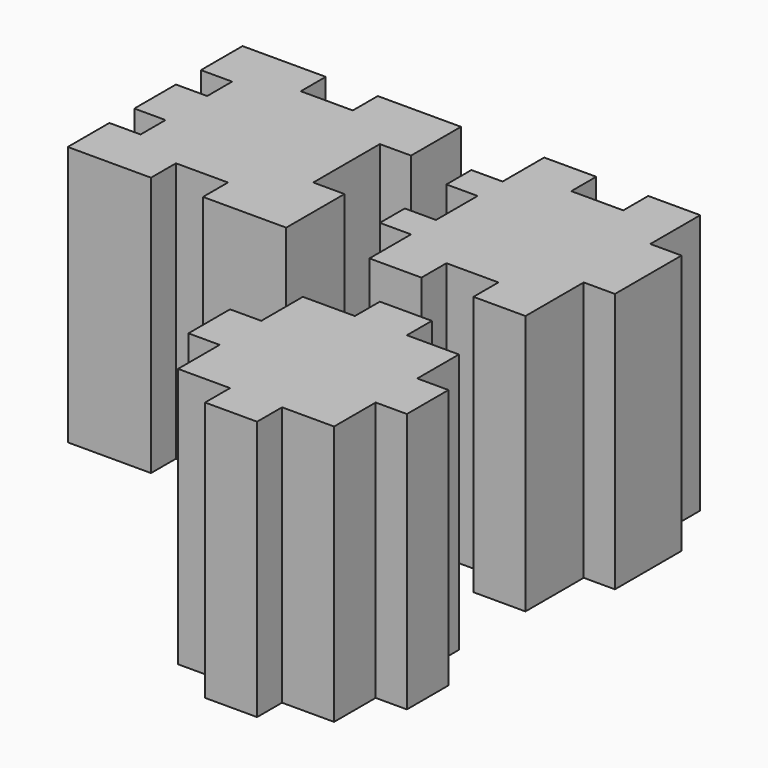
from build123d import *

# Parameters (mm, degrees)
F1_DEPTH = 25


# Not quite as in the source:
# - a feature names something its author has since deleted; it is built from what else it names


with BuildPart() as f1:
    # F0 (on Top) → F1 (new body)
    with BuildSketch(Plane.XY):
        Polygon((10.5, 10.5), (5.5, 10.5), (5.5, 5.5), (2.5, 5.5), (2.5, 2.5), (5.5, 2.5), (5.5, -2.5), (2.5, -2.5), (2.5, -5.5), (5.5, -5.5), (5.5, -10.5), (10.5, -10.5), (10.5, -7.5), (15.5, -7.5), (15.5, -10.5), (20.5, -10.5), (20.5, -3.5), (23.5, -3.5), (23.5, 4.5), (20.5, 4.5), (20.5, 10.5), (15.5, 10.5), (15.5, 7.5), (10.5, 7.5), align=None)
    extrude(amount=F1_DEPTH)


with BuildPart() as f1b:
    # F0 (on Top) → F1, piece 2 (new body)
    with BuildSketch(Plane.XY):
        Polygon((-15.5, 10.5), (-23.5, 10.5), (-23.5, 5.5), (-20.5, 5.5), (-20.5, 2.5), (-23.5, 2.5), (-23.5, -2.5), (-20.5, -2.5), (-20.5, -5.5), (-23.5, -5.5), (-23.5, -10.5), (-15.5, -10.5), (-15.5, -7.5), (-10.5, -7.5), (-10.5, -10.5), (-2.5, -10.5), (-2.5, -3.5), (-5.5, -3.5), (-5.5, 4.5), (-2.5, 4.5), (-2.5, 10.5), (-10.5, 10.5), (-10.5, 7.5), (-15.5, 7.5), align=None)
    extrude(amount=F1_DEPTH)


with BuildPart() as f1c:
    # F0 (on Top) → F1, piece 3 (new body)
    with BuildSketch(Plane.XY):
        Polygon((10.5, -18.5), (5.5, -18.5), (5.5, -23.5), (2.5, -23.5), (2.5, -28.5), (5.5, -28.5), (5.5, -33.5), (10.5, -33.5), (10.5, -36.5), (15.5, -36.5), (15.5, -33.5), (20.5, -33.5), (20.5, -28.5), (23.5, -28.5), (23.5, -23.5), (20.5, -23.5), (20.5, -18.5), (15.5, -18.5), (15.5, -15.5), (10.5, -15.5), align=None)
    extrude(amount=F1_DEPTH)


solid = Compound([f1.part, f1b.part, f1c.part])
